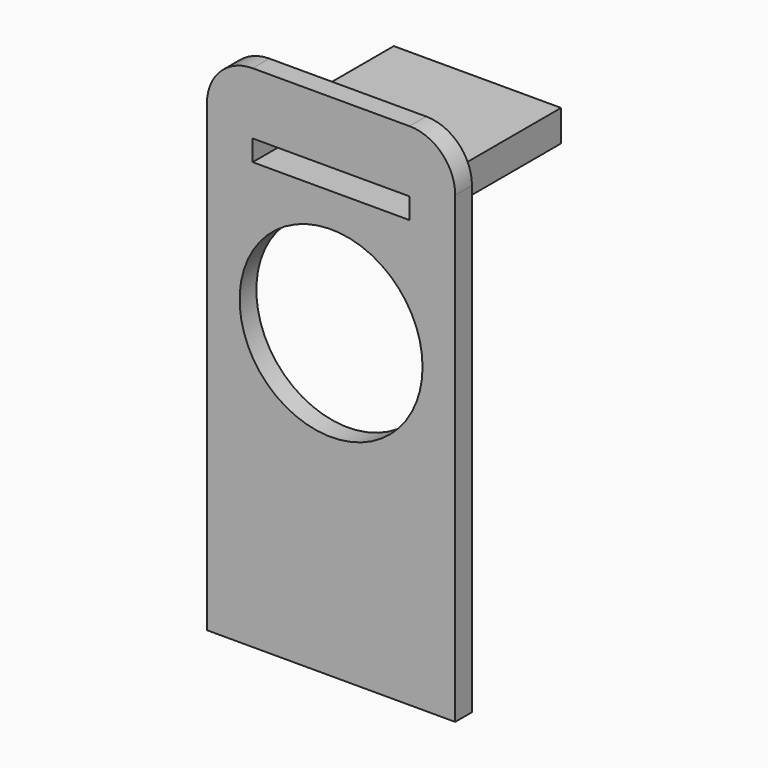
from build123d import *

# Parameters (mm, degrees)
F1_DEPTH  = 8
F2_R      = 35
F3_DEPTH  = 10
F4_W      = 30
F4_H      = 8
F5_DEPTH  = 8
F6_W      = 60
F6_H      = 2
F7_DEPTH  = 60
F8_W      = 64
F8_H      = 12
F9_DEPTH  = 2
F10_R     = 2.5
F11_DEPTH = 4


# Not quite as in the source:
# - the program builds the solid bodies; features that only make, move or delete a surface that nothing else refers to are left out


with BuildPart() as f1:
    # F0 (on Front) → F1 (new body)
    with BuildSketch(Plane.XZ):
        with BuildLine():
            Line((30, 44.5009035608), (-30, 44.5009035608))
            ThreePointArc((-30, 44.5009035608), (-42.3743686708, 39.3752722315), (-47.5, 27.0009035608))
            Line((-47.5, 27.0009035608), (-47.5, -150.4990964392))
            Line((-47.5, -150.4990964392), (47.5, -150.4990964392))
            Line((47.5, -150.4990964392), (47.5, 27.0009035608))
            ThreePointArc((47.5, 27.0009035608), (42.3743686708, 39.3752722315), (30, 44.5009035608))
        make_face()
    extrude(amount=F1_DEPTH)

    # F2 (on face) → F3 (cut)
    with BuildSketch(Plane.XZ.offset(8)):
        with Locations((0, -35)):
            Circle(F2_R)
    extrude(amount=-F3_DEPTH, mode=Mode.SUBTRACT)

    # F4 (on face) → F5 (cut)
    with BuildSketch(Plane.XZ.offset(8)):
        with Locations((-15, 16.8591848421)):
            Rectangle(F4_W, F4_H)
        with Locations((15, 16.8591848421)):
            Rectangle(F4_W, F4_H)
    extrude(amount=-F5_DEPTH, mode=Mode.SUBTRACT)

    # F6 (on face) → F7 (join)
    with BuildSketch(Plane(origin=(0, 0, 0), x_dir=(-1, 0, 0), z_dir=(0, 1, 0))):
        with Locations((0, 21.8591848421)):
            Rectangle(F6_W, F6_H)
        Polygon((-30, 12.8591848421), (-30, 20.8591848421), (-30, 22.8591848421), (-32, 22.8591848421), (-32, 10.8591848421), (-30, 10.8591848421), align=None)
        Polygon((30, 22.8591848421), (30, 20.8591848421), (30, 12.8591848421), (30, 10.8591848421), (32, 10.8591848421), (32, 22.8591848421), align=None)
        with Locations((0, 11.8591848421)):
            Rectangle(F6_W, F6_H)
    extrude(amount=F7_DEPTH)

    # F8 (on face) → F9 (join)
    with BuildSketch(Plane(origin=(0, 60, 0), x_dir=(-1, 0, 0), z_dir=(0, 1, 0))):
        with Locations((0, 16.8591848421)):
            Rectangle(F8_W, F8_H)
    extrude(amount=F9_DEPTH)

    # F10 (on face) → F11 (cut)
    with BuildSketch(Plane(origin=(0, 0, 10.8591848421), x_dir=(1, 0, 0), z_dir=(0, 0, -1))):
        with Locations((-24.5, -54.5)):
            Circle(F10_R)
    extrude(amount=-F11_DEPTH, mode=Mode.SUBTRACT)


solid = f1.part
